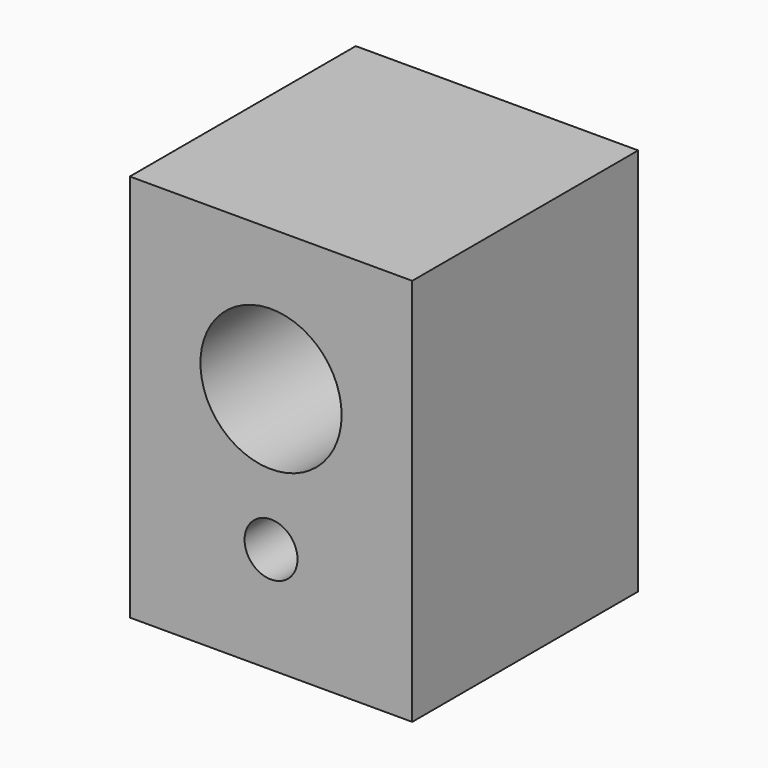
from build123d import *

# Parameters (mm, degrees)
F0_R     = 12.7
F1_DEPTH = 25.4


with BuildPart() as f1:
    # F0 (on Front) → F1 (new body, symmetric)
    with BuildSketch(Plane.XZ):
        Polygon((-12.7, -44.45), (0, -44.45), (12.7, -44.45), (25.4, -44.45), (25.4, 25.4), (-25.4, 25.4), (-25.4, -44.45), align=None)
        with BuildLine():
            ThreePointArc((0, -30.1625), (-3.3675960454, -22.0324039546), (4.7625, -25.4))
            ThreePointArc((4.7625, -25.4), (3.3675960454, -28.7675960454), (0, -30.1625))
        make_face(mode=Mode.SUBTRACT)
        Circle(F0_R, mode=Mode.SUBTRACT)
    extrude(amount=F1_DEPTH, both=True)

    # F0 (on Front) → F2 (revolve)
    with BuildSketch(Plane.XZ):
        Polygon((12.7, -44.45), (0, -44.45), (0, -50.8), (6.35, -50.8), (12.7, -50.8), align=None)
        Polygon((6.35, -50.8), (0, -50.8), (0, -53.34), (2.54, -53.34), (6.35, -53.34), align=None)
        Polygon((2.54, -53.34), (0, -53.34), (0, -57.15), align=None)
    revolve(axis=Axis((0, 0, -41.275), (0, 0, -1)))


solid = f1.part
